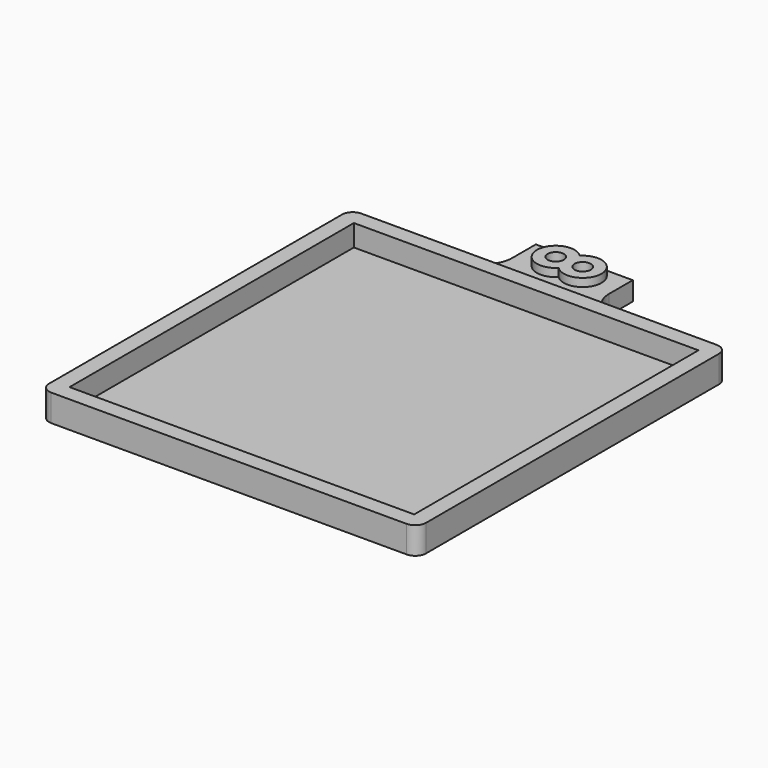
from build123d import *

# Parameters (mm, degrees)
F1_DEPTH = 5
F0_R     = 1.5
F2_DEPTH = 3.5
F3_DEPTH = 1
F4_R     = 2


# Not quite as in the source:
# - a feature names something its author has since deleted; it is built from what else it names


with BuildPart() as f1:
    # F0 (on Top) → F1 (new body)
    with BuildSketch(Plane.XY):
        Polygon((35, 36), (14, 36), (-14, 36), (-35, 36), (-35, -36), (35, -36), (35, -33), (35, 33), align=None)
        Polygon((-32, 14.5), (-32, 33), (32, 33), (32, -2), (32, -12.5), (32, -33), (12.7135775983, -33), (-8, -33), (-32, -33), (-32, -14), (-32, 10.5), align=None, mode=Mode.SUBTRACT)
    extrude(amount=F1_DEPTH)



with BuildPart() as f1b:
    # F0 (on Top) → F1, piece 2 (new body)
    with BuildSketch(Plane.XY):
        with BuildLine():
            ThreePointArc((0, 40.5505102572), (5.7267021942, 41.6441264992), (2.5, 46.5))
            ThreePointArc((2.5, 46.5), (1.1441264992, 46.2267021942), (0, 45.4494897428))
            ThreePointArc((0, 45.4494897428), (-1.1441264992, 46.2267021942), (-2.5, 46.5))
            ThreePointArc((-2.5, 46.5), (-5.7267021942, 41.6441264992), (0, 40.5505102572))
        make_face()
        with Locations((-2.5, 43)):
            Circle(F0_R, mode=Mode.SUBTRACT)
        with Locations((2.5, 43)):
            Circle(F0_R, mode=Mode.SUBTRACT)
    extrude(amount=F1_DEPTH)


with BuildPart() as f1_1:
    add(f1.part)

    add(f1b.part)  # F2 merges F1b
    # F0 (on Top) → F2 (join)
    with BuildSketch(Plane.XY):
        with BuildLine():
            Line((-14, 36), (14, 36))
            ThreePointArc((14, 36), (10.4644660941, 37.4644660941), (9, 41))
            Line((9, 41), (9, 46.5))
            Line((9, 46.5), (2.5, 46.5))
            ThreePointArc((2.5, 46.5), (5.7267021942, 41.6441264992), (0, 40.5505102572))
            ThreePointArc((0, 40.5505102572), (-5.7267021942, 41.6441264992), (-2.5, 46.5))
            Line((-2.5, 46.5), (-9, 46.5))
            Line((-9, 46.5), (-9, 41))
            ThreePointArc((-9, 41), (-10.4644660941, 37.4644660941), (-14, 36))
        make_face()
        with BuildLine():
            ThreePointArc((0, 45.4494897428), (1.1441264992, 46.2267021942), (2.5, 46.5))
            Line((2.5, 46.5), (-2.5, 46.5))
            ThreePointArc((-2.5, 46.5), (-1.1441264992, 46.2267021942), (0, 45.4494897428))
        make_face()
    extrude(amount=F2_DEPTH)

    # F0 (on Top) → F3 (join)
    with BuildSketch(Plane.XY):
        Polygon((32, 33), (-32, 33), (-32, 14.5), (-32, 10.5), (-32, -14), (-32, -33), (-8, -33), (12.7135775983, -33), (32, -33), (32, -12.5), (32, -2), align=None)
    extrude(amount=F3_DEPTH)

    # F4
    f4_edges = [f1_1.edges().sort_by_distance(p)[0] for p in [
        (-35, -36, 2.5),
        (35, -36, 2.5),
        (-35, 36, 2.5),
        (35, 36, 2.5),
    ]]
    fillet(f4_edges, radius=F4_R)


solid = f1_1.part
